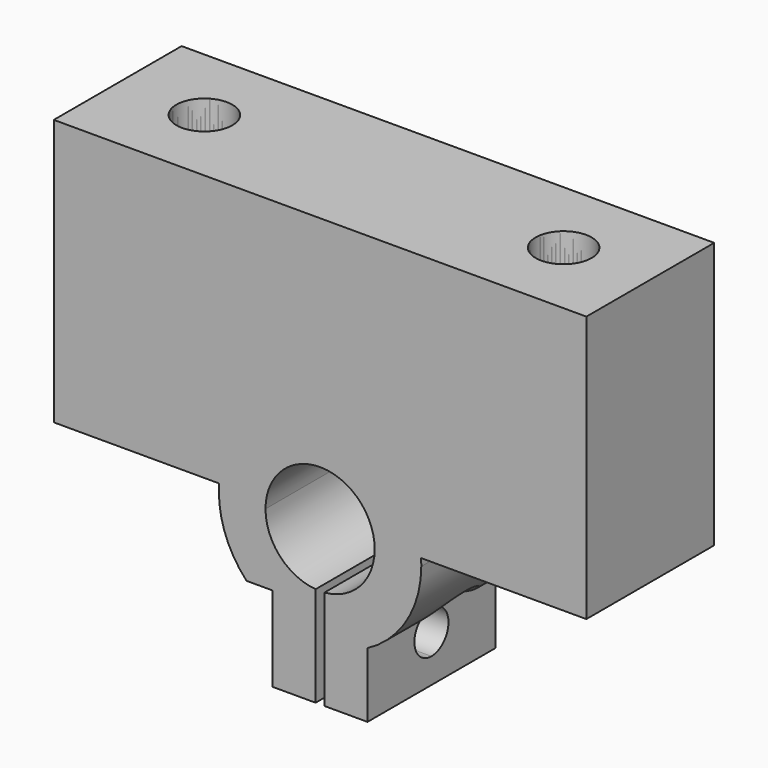
from build123d import *

# Parameters (mm, degrees)
F1_DEPTH  = 12
F3_DEPTH  = 25
F5_DEPTH  = 25
F7_DEPTH  = 25
F8_R      = 3.5
F9_DEPTH  = 25
F10_R     = 3.5
F11_DEPTH = 25
F12_DEPTH = 25
F13_W     = 40
F13_H     = 12
F13_R     = 2.1
F14_DEPTH = 7.55
F16_W     = 13.017164
F16_H     = 12
F16_R     = 2.1
F15_W     = 13.017164
F15_H     = 12
F15_R     = 2.1
F17_DEPTH = 2.45


with BuildPart() as f1:
    # F0 (on Front) → F1 (new body)
    with BuildSketch(Plane.XZ):
        with BuildLine():
            ThreePointArc((4.1, 0), (3.015615, -2.777781), (0.336066, -4.086204))
            Line((0.336066, -4.086204), (0.336066, -11.593204))
            Line((0.336066, -11.593204), (3.5625, -11.593204))
            Line((3.5625, -11.593204), (3.5625, -6.713315))
            ThreePointArc((3.5625, -6.713315), (6.512872, -3.91695), (7.6, 0))
            Line((7.6, 0), (4.1, 0))
        make_face()
        with BuildLine():
            ThreePointArc((2.794638, 3), (3.759522, 1.635846), (4.1, 0))
            Line((4.1, 0), (7.6, 0))
            ThreePointArc((7.6, 0), (7.44411, 1.531412), (6.982836, 3))
            Line((6.982836, 3), (2.794638, 3))
        make_face()
        with BuildLine():
            ThreePointArc((-2.794638, 3), (0, 4.1), (2.794638, 3))
            Line((2.794638, 3), (6.982836, 3))
            ThreePointArc((6.982836, 3), (0, 7.6), (-6.982836, 3))
            Line((-6.982836, 3), (-2.794638, 3))
        make_face()
        with BuildLine():
            ThreePointArc((-4.1, 0), (-3.759522, 1.635846), (-2.794638, 3))
            Line((-2.794638, 3), (-6.982836, 3))
            ThreePointArc((-6.982836, 3), (-7.44411, 1.531412), (-7.6, 0))
            Line((-7.6, 0), (-4.1, 0))
        make_face()
        with BuildLine():
            ThreePointArc((-6.982836, 3), (0, 7.6), (6.982836, 3))
            Line((6.982836, 3), (20, 3))
            Line((20, 3), (20, 13))
            Line((20, 13), (-20, 13))
            Line((-20, 13), (-20, 3))
            Line((-20, 3), (-6.982836, 3))
        make_face()
        with BuildLine():
            ThreePointArc((-0.336066, -4.086204), (-3.015615, -2.777781), (-4.1, 0))
            Line((-4.1, 0), (-7.6, 0))
            ThreePointArc((-7.6, 0), (-6.512872, -3.91695), (-3.5625, -6.713315))
            Line((-3.5625, -6.713315), (-3.5625, -11.593204))
            Line((-3.5625, -11.593204), (-0.336066, -11.593204))
            Line((-0.336066, -11.593204), (-0.336066, -4.086204))
        make_face()
    extrude(amount=F1_DEPTH)

    # F2 (on face) → F3 (cut)
    with BuildSketch(Plane(origin=(0, 0, 3), x_dir=(1, 0, 0), z_dir=(0, 0, -1))):
        with BuildLine():
            ThreePointArc((-11.391418, 6), (-12.006494, 7.484924), (-13.491418, 8.1))
            Line((-13.491418, 8.1), (-13.491418, 3.9))
            ThreePointArc((-13.491418, 3.9), (-12.006494, 4.515076), (-11.391418, 6))
        make_face()
        with BuildLine():
            Line((-13.491418, 3.9), (-13.491418, 8.1))
            ThreePointArc((-13.491418, 8.1), (-15.591418, 6), (-13.491418, 3.9))
        make_face()
    extrude(amount=-F3_DEPTH, mode=Mode.SUBTRACT)

    # F4 (on face) → F5 (cut)
    with BuildSketch(Plane(origin=(0, 0, 3), x_dir=(1, 0, 0), z_dir=(0, 0, -1))):
        with BuildLine():
            ThreePointArc((15.591418, 6), (14.976342, 7.484924), (13.491418, 8.1))
            Line((13.491418, 8.1), (13.491418, 3.9))
            ThreePointArc((13.491418, 3.9), (14.976342, 4.515076), (15.591418, 6))
        make_face()
        with BuildLine():
            Line((13.491418, 3.9), (13.491418, 8.1))
            ThreePointArc((13.491418, 8.1), (11.391418, 6), (13.491418, 3.9))
        make_face()
    extrude(amount=-F5_DEPTH, mode=Mode.SUBTRACT)

    # F6 (on face) → F7 (cut)
    with BuildSketch(Plane(origin=(-3.5625, 0, 0), x_dir=(0, -1, 0), z_dir=(-1, 0, 0))):
        with BuildLine():
            ThreePointArc((6, -6.493204), (4.4, -8.093204), (6, -9.693204))
            Line((6, -9.693204), (6, -6.493204))
        make_face()
        with BuildLine():
            Line((6, -6.493204), (6, -9.693204))
            ThreePointArc((6, -9.693204), (7.131371, -9.224574), (7.6, -8.093204))
            ThreePointArc((7.6, -8.093204), (7.131371, -6.961833), (6, -6.493204))
        make_face()
    extrude(amount=-F7_DEPTH, mode=Mode.SUBTRACT)

    # F8 (on face) → F9 (cut)
    with BuildSketch(Plane(origin=(-3.5625, 0, 0), x_dir=(0, -1, 0), z_dir=(-1, 0, 0))):
        with Locations((10, -8.093204)):
            Circle(F8_R)
    extrude(amount=F9_DEPTH, mode=Mode.SUBTRACT)

    # F10 (on face) → F11 (cut)
    with BuildSketch(Plane.YZ.offset(3.5625)):
        with Locations((-6, -8.093204)):
            Circle(F10_R)
    extrude(amount=F11_DEPTH, mode=Mode.SUBTRACT)

    # F8 (on face) → F12 (cut)
    with BuildSketch(Plane(origin=(-3.5625, 0, 0), x_dir=(0, -1, 0), z_dir=(-1, 0, 0))):
        with Locations((10, -8.093204)):
            Circle(F8_R)
    extrude(amount=F12_DEPTH, mode=Mode.SUBTRACT)

    # F13 (on face) → F14 (join)
    with BuildSketch(Plane.XY.offset(13)):
        with Locations((0, -6)):
            Rectangle(F13_W, F13_H)
        with Locations((-13.491418, -6)):
            Circle(F13_R, mode=Mode.SUBTRACT)
        with Locations((13.491418, -6)):
            Circle(F13_R, mode=Mode.SUBTRACT)
    extrude(amount=F14_DEPTH)

    # F16 (on face) + F15 (on face) → F17 (join)
    with BuildSketch(Plane(origin=(0, 0, 3), x_dir=(1, 0, 0), z_dir=(0, 0, -1))):
        with Locations((13.491418, 6)):
            Rectangle(F16_W, F16_H)
        with Locations((13.491418, 6)):
            Circle(F16_R, mode=Mode.SUBTRACT)
    with BuildSketch(Plane(origin=(0, 0, 3), x_dir=(1, 0, 0), z_dir=(0, 0, -1))):
        with Locations((-13.491418, 6)):
            Rectangle(F15_W, F15_H)
        with Locations((-13.491418, 6)):
            Circle(F15_R, mode=Mode.SUBTRACT)
    extrude(amount=F17_DEPTH)


with BuildPart() as f18_1:
    # F18: copy of F1
    add(f1.part)


solid = Compound([f1.part, f18_1.part])
